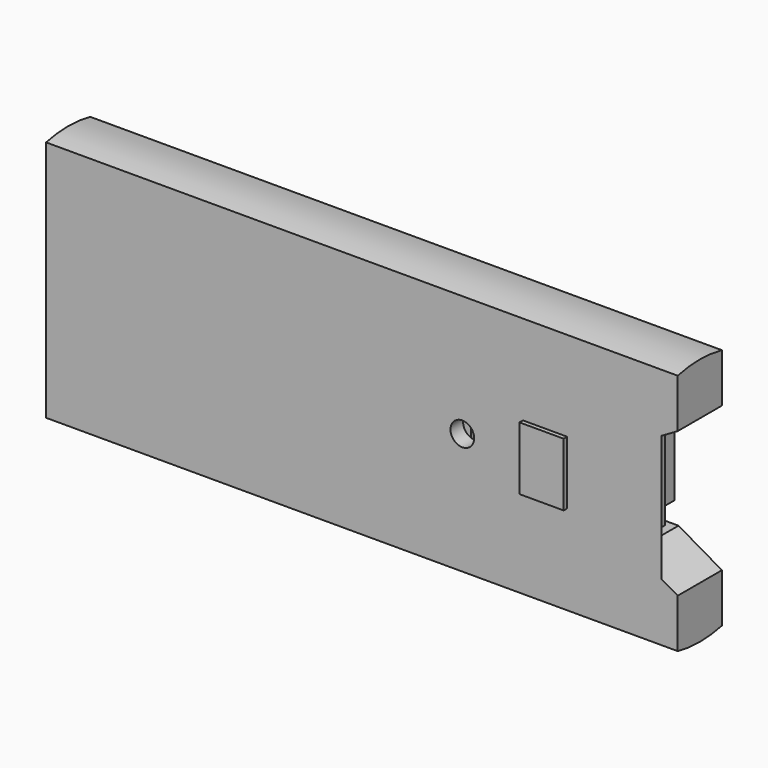
from build123d import *

# Parameters (mm, degrees)
F0_W      = 36
F0_H      = 12.4
F0_R      = 1.1
F0_W_2    = 4.4
F0_H_2    = 7.8
F0_W_3    = 12.5
F0_H_3    = 11
F1_DEPTH  = 1.55
F2_DEPTH  = 2
F0_W_4    = 1.15
F3_DEPTH  = 2.9
F0_W_5    = 3.5
F4_DEPTH  = 1.5
F5_DEPTH  = 1.3
F6_R      = 1
F7_DEPTH  = 3
F8_W      = 5.6
F8_H      = 8
F10_DEPTH = 4.5
F9_W      = 1.5
F9_H      = 10
F11_DEPTH = 1.4
F9_W_2    = 6.5
F12_DEPTH = 2.5
F13_W     = 80
F13_H     = 35
F14_DEPTH = 7
F15_W     = 7
F15_H     = 10
F16_DEPTH = 2
F15_W_2   = 4
F15_H_2   = 1.5
F17_DEPTH = 5.45
F18_DEPTH = 3.95
F19_R     = 1.5
F20_DEPTH = 2
F21_W     = 5
F21_H     = 12
F22_DEPTH = 5.5
F22_TAPER = -30
F24_DEPTH = 80


with BuildPart() as f1:
    # F0 (on Front) → F1 (new body)
    with BuildSketch(Plane.XZ):
        Polygon((-30.5, -8.95), (30.5, -8.95), (30.5, -5.5), (18, -5.5), (18, 5.5), (30.5, 5.5), (30.5, 8.95), (-30.5, 8.95), (-30.5, 3.9), (-26.1, 3.9), (-26.1, -3.9), (-30.5, -3.9), align=None)
        with Locations((-7.5, 0)):
            Rectangle(F0_W, F0_H, mode=Mode.SUBTRACT)
        with Locations((12.72, 0)):
            Circle(F0_R, mode=Mode.SUBTRACT)
        with Locations((-28.3, 0)):
            Rectangle(F0_W_2, F0_H_2)
        with Locations((24.25, 0)):
            Rectangle(F0_W_3, F0_H_3)
        with Locations((12.72, 0)):
            Circle(F0_R)
        with Locations((-7.5, 0)):
            Rectangle(F0_W, F0_H)
    extrude(amount=-F1_DEPTH)

    # F0 (on Front) → F2 (join)
    with BuildSketch(Plane.XZ):
        with Locations((12.72, 0)):
            Circle(F0_R)
    extrude(amount=F2_DEPTH)

    # F0 (on Front) → F3 (join)
    with BuildSketch(Plane.XZ):
        with Locations((-28.3, 0)):
            Rectangle(F0_W_2, F0_H_2)
        with Locations((-31.075, 0)):
            Rectangle(F0_W_4, F0_H_2)
    extrude(amount=F3_DEPTH)

    # F0 (on Front) → F4 (join)
    with BuildSketch(Plane.XZ):
        with Locations((32.25, 0)):
            Rectangle(F0_W_5, F0_H_3)
        with Locations((24.25, 0)):
            Rectangle(F0_W_3, F0_H_3)
    extrude(amount=F4_DEPTH)

    # F0 (on Front) → F5 (join)
    with BuildSketch(Plane.XZ):
        with Locations((-7.5, 0)):
            Rectangle(F0_W, F0_H)
    extrude(amount=F5_DEPTH)

    # F6 (on face) → F7 (join)
    with BuildSketch(Plane(origin=(0, 1.55, 0), x_dir=(-1, 0, 0), z_dir=(0, 1, 0))):
        with Locations((29.21, -7.62)):
            Circle(F6_R)
        with Locations((29.21, 7.62)):
            Circle(F6_R)
        with Locations((26.67, -7.62)):
            Circle(F6_R)
        with Locations((26.67, 7.62)):
            Circle(F6_R)
        with Locations((24.13, -7.62)):
            Circle(F6_R)
        with Locations((24.13, 7.62)):
            Circle(F6_R)
        with Locations((21.59, -7.62)):
            Circle(F6_R)
        with Locations((21.59, 7.62)):
            Circle(F6_R)
        with Locations((19.05, -7.62)):
            Circle(F6_R)
        with Locations((19.05, 7.62)):
            Circle(F6_R)
        with Locations((16.51, -7.62)):
            Circle(F6_R)
        with Locations((16.51, 7.62)):
            Circle(F6_R)
        with Locations((13.97, -7.62)):
            Circle(F6_R)
        with Locations((13.97, 7.62)):
            Circle(F6_R)
        with Locations((11.43, -7.62)):
            Circle(F6_R)
        with Locations((11.43, 7.62)):
            Circle(F6_R)
        with Locations((8.89, -7.62)):
            Circle(F6_R)
        with Locations((8.89, 7.62)):
            Circle(F6_R)
        with Locations((6.35, -7.62)):
            Circle(F6_R)
        with Locations((6.35, 7.62)):
            Circle(F6_R)
        with Locations((3.81, -7.62)):
            Circle(F6_R)
        with Locations((3.81, 7.62)):
            Circle(F6_R)
        with Locations((1.27, -7.62)):
            Circle(F6_R)
        with Locations((1.27, 7.62)):
            Circle(F6_R)
        with Locations((-1.27, -7.62)):
            Circle(F6_R)
        with Locations((-1.27, 7.62)):
            Circle(F6_R)
        with Locations((-3.81, -7.62)):
            Circle(F6_R)
        with Locations((-3.81, 7.62)):
            Circle(F6_R)
        with Locations((-6.35, -7.62)):
            Circle(F6_R)
        with Locations((-6.35, 7.62)):
            Circle(F6_R)
        with Locations((-8.89, -7.62)):
            Circle(F6_R)
        with Locations((-8.89, 7.62)):
            Circle(F6_R)
        with Locations((-11.43, -7.62)):
            Circle(F6_R)
        with Locations((-11.43, 7.62)):
            Circle(F6_R)
        with Locations((-13.97, -7.62)):
            Circle(F6_R)
        with Locations((-13.97, 7.62)):
            Circle(F6_R)
        with Locations((-16.51, -7.62)):
            Circle(F6_R)
        with Locations((-16.51, 7.62)):
            Circle(F6_R)
        with Locations((-19.05, -7.62)):
            Circle(F6_R)
        with Locations((-19.05, 7.62)):
            Circle(F6_R)
        with Locations((-21.59, -7.62)):
            Circle(F6_R)
        with Locations((-21.59, 7.62)):
            Circle(F6_R)
        with Locations((-24.13, -7.62)):
            Circle(F6_R)
        with Locations((-24.13, 7.62)):
            Circle(F6_R)
        with Locations((-26.67, -7.62)):
            Circle(F6_R)
        with Locations((-26.67, 7.62)):
            Circle(F6_R)
        with Locations((-29.21, -7.62)):
            Circle(F6_R)
        with Locations((-29.21, 7.62)):
            Circle(F6_R)
    extrude(amount=F7_DEPTH)


with BuildPart() as f10:
    # F8 (on face) → F10 (new body)
    with BuildSketch(Plane.XZ.offset(1.5)):
        with Locations((23.2, 0)):
            Rectangle(F8_W, F8_H)
    extrude(amount=F10_DEPTH)


with BuildPart() as f11:
    # F9 (on face) → F11 (new body)
    with BuildSketch(Plane(origin=(0, 1.55, 0), x_dir=(-1, 0, 0), z_dir=(0, 1, 0))):
        with Locations((-31.25, 0)):
            Rectangle(F9_W, F9_H)
    extrude(amount=-F11_DEPTH)

    # F9 (on face) → F12 (join)
    with BuildSketch(Plane(origin=(0, 1.55, 0), x_dir=(-1, 0, 0), z_dir=(0, 1, 0))):
        with Locations((-31.25, 0)):
            Rectangle(F9_W, F9_H)
        with Locations((-27.25, 0)):
            Rectangle(F9_W_2, F9_H)
    extrude(amount=F12_DEPTH)


with BuildPart() as f14:
    # F13 (on face) → F14 (new body)
    with BuildSketch(Plane(origin=(0, 1.55, 0), x_dir=(-1, 0, 0), z_dir=(0, 1, 0))):
        Rectangle(F13_W, F13_H)
        Polygon((-34.5, 6), (-31, 6), (-31, 9.45), (31, 9.45), (31, 4.4), (32.15, 4.4), (32.15, -4.4), (31, -4.4), (31, -9.45), (-31, -9.45), (-31, -6), (-34.5, -6), align=None, mode=Mode.SUBTRACT)
    extrude(amount=-F14_DEPTH)

    # F15 (on face) → F16 (join)
    with BuildSketch(Plane.XZ.offset(5.45)):
        Polygon((-31, 9.45), (-31, 6.1), (-27, 6.1), (-27, 4.6), (-31, 4.6), (-31, 4.4), (-32.15, 4.4), (-32.15, -4.4), (-31, -4.4), (-31, -4.6), (-27, -4.6), (-27, -6.1), (-31, -6.1), (-31, -9.45), (31, -9.45), (31, -6), (34.5, -6), (34.5, 6), (31, 6), (31, 9.45), align=None)
        with Locations((26.5, 0)):
            Rectangle(F15_W, F15_H, mode=Mode.SUBTRACT)
    extrude(amount=-F16_DEPTH)

    # F15 (on face) → F17 (join, through all)
    with BuildSketch(Plane.XZ.offset(5.45)):
        with Locations((-29, 5.35)):
            Rectangle(F15_W_2, F15_H_2)
        with Locations((-29, -5.35)):
            Rectangle(F15_W_2, F15_H_2)
    extrude(amount=-F17_DEPTH)

    # F15 (on face) → F18 (join, through all)
    with BuildSketch(Plane.XZ.offset(5.45)):
        with Locations((26.5, 0)):
            Rectangle(F15_W, F15_H)
    extrude(amount=-F18_DEPTH)

    # F19 (on face) → F20 (cut, through all)
    with BuildSketch(Plane.XZ.offset(5.45)):
        with Locations((12.72, 0)):
            Circle(F19_R)
    extrude(amount=-F20_DEPTH, mode=Mode.SUBTRACT)

    # F21 (on face) → F22 (cut, through all)
    with BuildSketch(Plane(origin=(34.5, 0, 0), x_dir=(0, -1, 0), z_dir=(-1, 0, 0))):
        with Locations((0.95, 0)):
            Rectangle(F21_W, F21_H)
    extrude(amount=-F22_DEPTH, taper=F22_TAPER, mode=Mode.SUBTRACT)

    # F23 (on face) → F24 (cut)
    with BuildSketch(Plane(origin=(-40, 0, 0), x_dir=(0, -1, 0), z_dir=(-1, 0, 0))):
        with BuildLine():
            ThreePointArc((5.45, -15.3561876779), (1.95, -15.75), (-1.55, -15.3561876779))
            Line((-1.55, -15.3561876779), (-1.55, -17.5))
            Line((-1.55, -17.5), (5.45, -17.5))
            Line((5.45, -17.5), (5.45, -15.3561876779))
        make_face()
        with BuildLine():
            Line((5.45, 17.5), (-1.55, 17.5))
            Line((-1.55, 17.5), (-1.55, 15.3561876779))
            ThreePointArc((-1.55, 15.3561876779), (1.95, 15.75), (5.45, 15.3561876779))
            Line((5.45, 15.3561876779), (5.45, 17.5))
        make_face()
    extrude(amount=-F24_DEPTH, mode=Mode.SUBTRACT)


solid = Compound([f1.part, f10.part, f11.part, f14.part])
